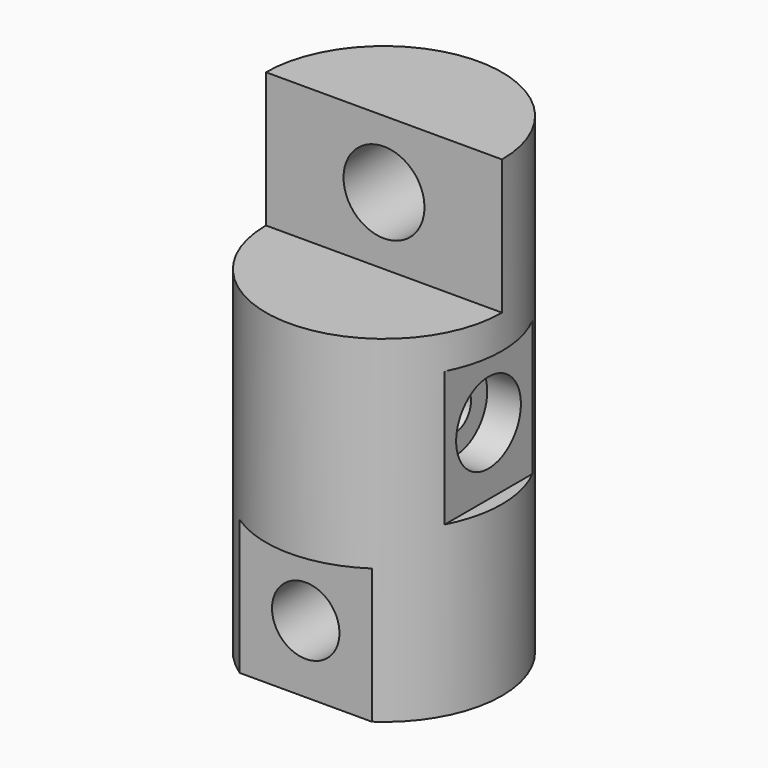
from build123d import *

# Parameters (mm, degrees)
F0_W            = 17.5
F0_H            = 70
F2_W            = 17.5
F2_H            = 20
F3_DEPTH        = 17.501
F3_DEPTH_BACK   = 17.501
F5_D            = 12
F7_START        = 14.5
F6_W            = 35
F6_H            = 20
F7_DEPTH        = 3.0010001
F9_D            = 10
F10_W           = 2
F10_H           = 20
F11_DEPTH       = 17.5010001
F11_DEPTH_BACK  = 17.5010001
F13_D           = 6
F13_CBORE_D     = 12
F13_CBORE_DEPTH = 5


# Not quite as in the source:
# - a pattern or mirror of a feature is missing from the dataset's text; its kind, count and spacing are read off the source's solid


with BuildPart() as f1:
    # F0 (on Front) → F1 (revolve)
    with BuildSketch(Plane.XZ):
        with Locations((8.75, 35)):
            Rectangle(F0_W, F0_H)
    revolve(axis=Axis((0, 0, 35), (0, 0, -1)))

    # F2 (on Right) → F3 (cut, two sides)
    with BuildSketch(Plane.YZ) as f3_sk:
        with Locations((-8.75, 60)):
            Rectangle(F2_W, F2_H)
    extrude(amount=-F3_DEPTH, mode=Mode.SUBTRACT)
    extrude(f3_sk.sketch, amount=F3_DEPTH_BACK, mode=Mode.SUBTRACT)

    # F5 (through all)
    with Locations(Plane.XZ):
        with Locations((0, 60)):
            Hole(F5_D / 2)

    # F6 (on Front) → F7 (cut)
    with BuildSketch(Plane.XZ.offset(F7_START)):
        with Locations((0, 10)):
            Rectangle(F6_W, F6_H)
    extrude(amount=F7_DEPTH, mode=Mode.SUBTRACT)

    # F9 (through all)
    with Locations(Plane.XZ.offset(14.5)):
        with Locations((0, 10)):
            Hole(F9_D / 2)

    # F10 (on Front) → F11 (cut, two sides)
    with BuildSketch(Plane.XZ) as f11_sk:
        with Locations((-16.5, 35)):
            Rectangle(F10_W, F10_H)
        with Locations((16.5, 35)):
            Rectangle(F10_W, F10_H)
    extrude(amount=-F11_DEPTH, mode=Mode.SUBTRACT)
    extrude(f11_sk.sketch, amount=F11_DEPTH_BACK, mode=Mode.SUBTRACT)

    # F13 (through all)
    with Locations(Plane.YZ.offset(15.5)):
        with Locations((0, 35)):
            f13 = CounterBoreHole(F13_D / 2, F13_CBORE_D / 2, F13_CBORE_DEPTH)

    # F13_copies: F13 across plane
    add(f13.mirror(Plane(origin=(0, 0, 0), x_dir=(0, 0, -1), z_dir=(-1, 0, 0))), mode=Mode.SUBTRACT)


solid = f1.part
